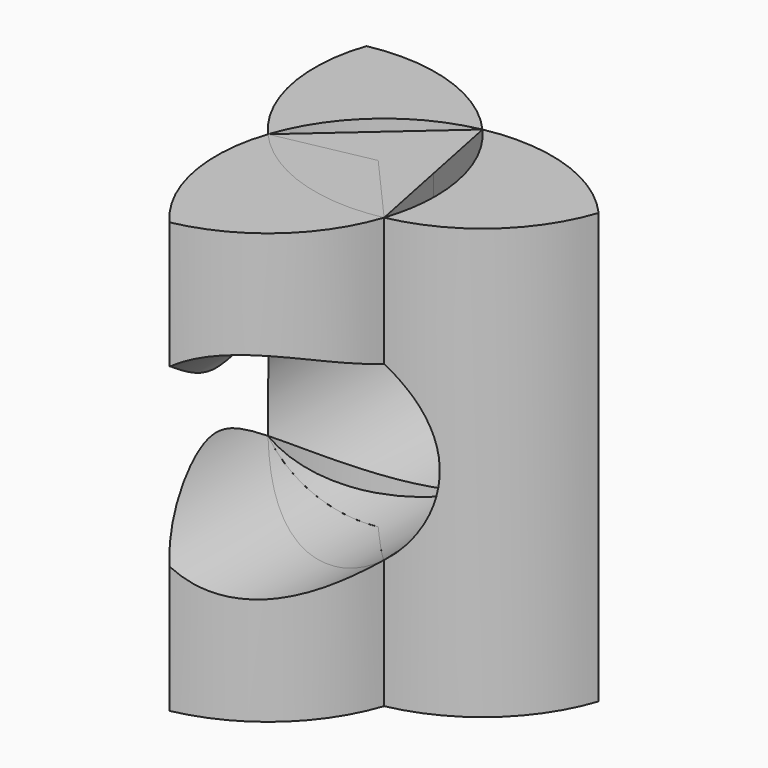
from build123d import *

# Parameters (mm, degrees)
F1_DEPTH = 10
F2_DEPTH = 10
F3_R     = 2.5
F4_DEPTH = 12.5


# Not quite as in the source:
# - a feature names something its author has since deleted; it is built from what else it names


with BuildPart() as f1:
    # F0 (on Top) → F1 (new body)
    with BuildSketch(Plane.XY):
        with BuildLine():
            ThreePointArc((-1.4366696316, -4.2673496606), (0.3714320322, -3.3700600464), (1.4886491985, -1.6889336141))
            ThreePointArc((1.4886491985, -1.6889336141), (-0.525857582, -1.5619583826), (-2.2069840144, -0.4447412162))
            ThreePointArc((-2.2069840144, -0.4447412162), (-2.3339592458, -2.4592479968), (-1.4366696316, -4.2673496606))
        make_face()
    extrude(amount=F1_DEPTH)


with BuildPart() as f1b:
    # F0 (on Top) → F1, piece 2 (new body)
    with BuildSketch(Plane.XY):
        with BuildLine():
            ThreePointArc((-2.2069840144, -0.4447412162), (-1.089766848, 1.2363852161), (0.7183348158, 2.1336748303))
            ThreePointArc((0.7183348158, 2.1336748303), (-0.9627916165, 3.2508919967), (-2.9772983971, 3.3778672281))
            ThreePointArc((-2.9772983971, 3.3778672281), (-3.1042736285, 1.3633604476), (-2.2069840144, -0.4447412162))
        make_face()
    extrude(amount=F1_DEPTH)


with BuildPart() as f1c:
    # F0 (on Top) → F1, piece 3 (new body)
    with BuildSketch(Plane.XY):
        with BuildLine():
            ThreePointArc((0.7183348158, 2.1336748303), (1.4408137839, 0.9334063774), (1.6924671736, -0.4447412162))
            ThreePointArc((1.6924671736, -0.4447412162), (1.6411753437, -1.0751292891), (1.4886491985, -1.6889336141))
            ThreePointArc((1.4886491985, -1.6889336141), (3.2967508623, -0.7916439999), (4.4139680287, 0.8894824325))
            ThreePointArc((4.4139680287, 0.8894824325), (2.7328415964, 2.0066995988), (0.7183348158, 2.1336748303))
        make_face()
    extrude(amount=F1_DEPTH)


with BuildPart() as f1d:
    # F0 (on Top) → F1, piece 4 (new body)
    with BuildSketch(Plane.XY):
        Polygon((0, 0), (1.4886491985, -1.6889336141), (1.1034920072, 0.2223706081), align=None)
        Polygon((1.1034920072, 0.2223706081), (0.7183348158, 2.1336748303), (0, 0), align=None)
        Polygon((0, 0), (0.7183348158, 2.1336748303), (-0.7443245993, 0.844466807), align=None)
        Polygon((-0.7443245993, 0.844466807), (-2.2069840144, -0.4447412162), (0, 0), align=None)
    extrude(amount=F1_DEPTH)


with BuildPart() as f2:
    # F0 (on Top) → F2 (new body, through all)
    with BuildSketch(Plane.XY):
        with BuildLine():
            ThreePointArc((-2.2069840144, -0.4447412162), (-0.525857582, -1.5619583826), (1.4886491985, -1.6889336141))
            Line((1.4886491985, -1.6889336141), (0, 0))
            Line((0, 0), (-2.2069840144, -0.4447412162))
        make_face()
    extrude(amount=F2_DEPTH)


with BuildPart() as f4_tool:
    # F3 (on Front) → F4 (new body, symmetric)
    with BuildSketch(Plane.XZ):
        with Locations((0, 5)):
            Circle(F3_R)
    extrude(amount=F4_DEPTH, both=True)


with BuildPart() as f1_1:
    add(f1.part)

    # F4: cut by f4_tool
    add(f4_tool.part, mode=Mode.SUBTRACT)


with BuildPart() as f1b_1:
    add(f1b.part)

    # F4: cut by f4_tool
    add(f4_tool.part, mode=Mode.SUBTRACT)


with BuildPart() as f1c_1:
    add(f1c.part)

    # F4: cut by f4_tool
    add(f4_tool.part, mode=Mode.SUBTRACT)


with BuildPart() as f1d_1:
    add(f1d.part)

    # F4: cut by f4_tool
    add(f4_tool.part, mode=Mode.SUBTRACT)


with BuildPart() as f2_1:
    add(f2.part)

    # F4: cut by f4_tool
    add(f4_tool.part, mode=Mode.SUBTRACT)


solid = Compound([f1_1.part, f1b_1.part, f1c_1.part, f1d_1.part, f2_1.part])
